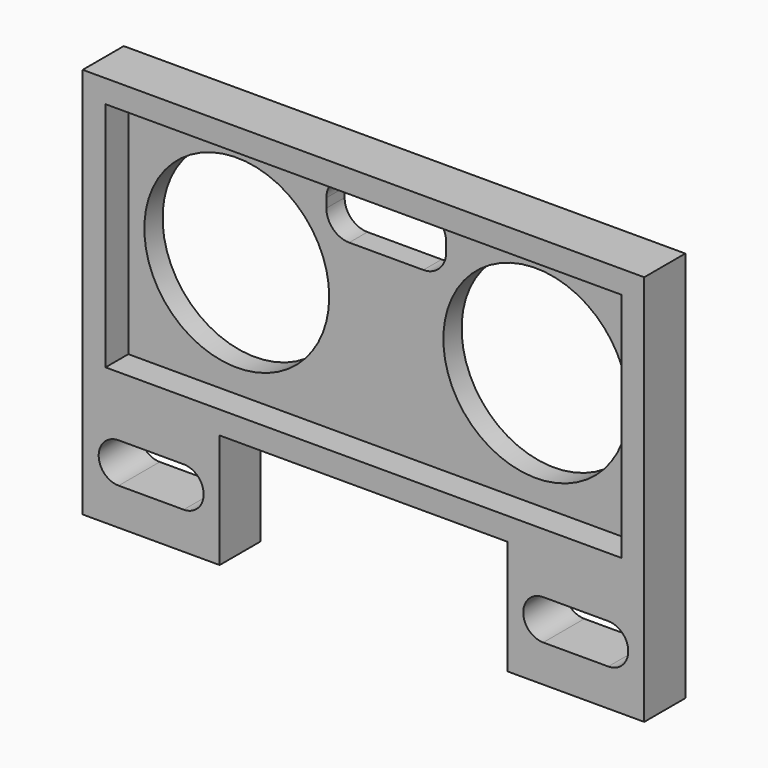
from build123d import *

# Parameters (mm, degrees)
F0_W     = 45.2
F0_H     = 20.3
F0_R     = 8.1
F0_W_2   = 10.5
F0_H_2   = 4.8
F1_DEPTH = 2
F0_W_3   = 12
F0_H_3   = 10
F2_DEPTH = 4.5
F3_R     = 2


# Not quite as in the source:
# - a feature names something its author has since deleted; it is built from what else it names


with BuildPart() as f1:
    # F0 (on Front) → F1 (new body)
    with BuildSketch(Plane.XZ):
        with Locations((0.3735902304, 3.0706598967)):
            Rectangle(F0_W, F0_H)
        with Locations((-12.7264097696, 3.0706598967)):
            Circle(F0_R, mode=Mode.SUBTRACT)
        with Locations((0.3735902304, 10.2206598967)):
            Rectangle(F0_W_2, F0_H_2, mode=Mode.SUBTRACT)
        with Locations((13.4735902304, 3.0706598967)):
            Circle(F0_R, mode=Mode.SUBTRACT)
    extrude(amount=F1_DEPTH)



with BuildPart() as f1b:
    # F0 (on Front) → F1, piece 2 (new body)
    with BuildSketch(Plane.XZ):
        with Locations((18.9735902304, -14.0793401033)):
            Rectangle(F0_W_3, F0_H_3)
        with BuildLine():
            ThreePointArc((16.1235902304, -15.8293401033), (14.3735902304, -14.0793401033), (16.1235902304, -12.3293401033))
            Line((16.1235902304, -12.3293401033), (21.8235902304, -12.3293401033))
            ThreePointArc((21.8235902304, -12.3293401033), (23.0610270975, -12.8419032362), (23.5735902304, -14.0793401033))
            ThreePointArc((23.5735902304, -14.0793401033), (23.0610270975, -15.3167769703), (21.8235902304, -15.8293401033))
            Line((21.8235902304, -15.8293401033), (16.1235902304, -15.8293401033))
        make_face(mode=Mode.SUBTRACT)
    extrude(amount=F1_DEPTH)


with BuildPart() as f1_1:
    add(f1.part)

    add(f1b.part)  # F2 merges F1b
    # F0 (on Front) → F2 (join)
    with BuildSketch(Plane.XZ):
        Polygon((24.9735902304, 15.2206598967), (-24.2264097696, 15.2206598967), (-24.2264097696, -9.0793401033), (-12.2264097696, -9.0793401033), (12.9735902304, -9.0793401033), (24.9735902304, -9.0793401033), align=None)
        with Locations((0.3735902304, 3.0706598967)):
            Rectangle(F0_W, F0_H, mode=Mode.SUBTRACT)
        with Locations((-18.2264097696, -14.0793401033)):
            Rectangle(F0_W_3, F0_H_3)
        with BuildLine():
            Line((-21.0764097696, -12.3293401033), (-15.3764097696, -12.3293401033))
            ThreePointArc((-15.3764097696, -12.3293401033), (-14.1389729025, -12.8419032362), (-13.6264097696, -14.0793401033))
            ThreePointArc((-13.6264097696, -14.0793401033), (-14.1389729025, -15.3167769703), (-15.3764097696, -15.8293401033))
            Line((-15.3764097696, -15.8293401033), (-21.0764097696, -15.8293401033))
            ThreePointArc((-21.0764097696, -15.8293401033), (-22.8264097696, -14.0793401033), (-21.0764097696, -12.3293401033))
        make_face(mode=Mode.SUBTRACT)
        with Locations((18.9735902304, -14.0793401033)):
            Rectangle(F0_W_3, F0_H_3)
        with BuildLine():
            ThreePointArc((16.1235902304, -15.8293401033), (14.3735902304, -14.0793401033), (16.1235902304, -12.3293401033))
            Line((16.1235902304, -12.3293401033), (21.8235902304, -12.3293401033))
            ThreePointArc((21.8235902304, -12.3293401033), (23.0610270975, -12.8419032362), (23.5735902304, -14.0793401033))
            ThreePointArc((23.5735902304, -14.0793401033), (23.0610270975, -15.3167769703), (21.8235902304, -15.8293401033))
            Line((21.8235902304, -15.8293401033), (16.1235902304, -15.8293401033))
        make_face(mode=Mode.SUBTRACT)
    extrude(amount=F2_DEPTH)

    # F3
    f3_edges = [f1_1.edges().sort_by_distance(p)[0] for p in [
        (-4.87641, -1, 7.82066),
        (-4.87641, -1, 12.62066),
        (5.62359, -1, 12.62066),
        (5.62359, -1, 7.82066),
    ]]
    fillet(f3_edges, radius=F3_R)


solid = f1_1.part
